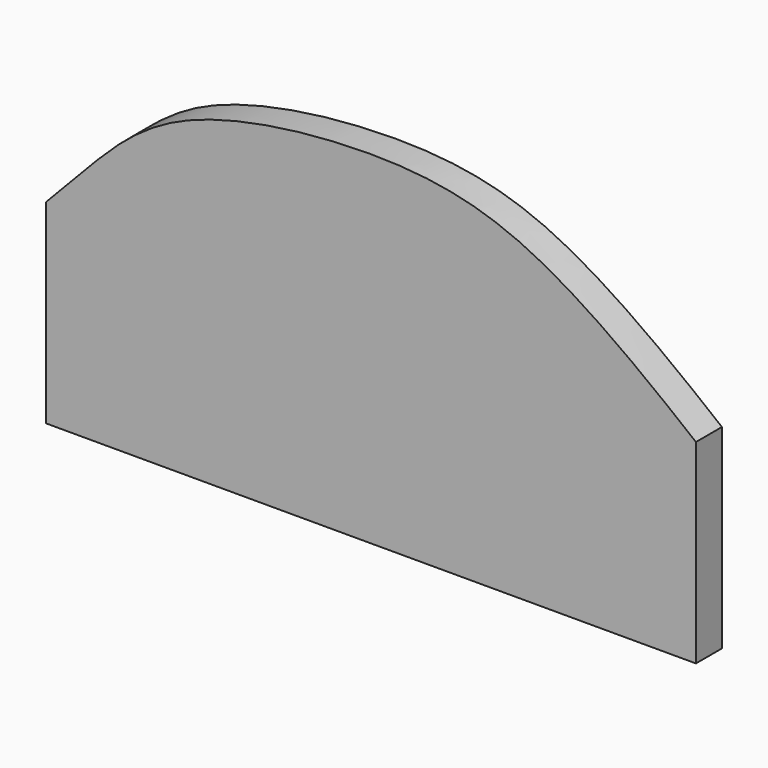
from build123d import *

# Parameters (mm, degrees)
F1_DEPTH = 6.35


with BuildPart() as f1:
    # F0 (on Front) → F1 (new body)
    with BuildSketch(Plane.XZ):
        with BuildLine():
            Line((-63.5, -38.1), (63.5, -38.1))
            Line((63.5, -38.1), (63.5, 0))
            add(Edge.make_bspline(
                [(-63.5, 0), (-60.67212487, 3.0032077004), (-54.227297491, 9.8476242046), (-38.4935463186, 25.5058577681), (0.6281666855, 30.5713039167), (28.1408073024, 25.8822175031), (51.7311119878, 9.4765375074), (60.0037451352, 2.8152524119), (63.5, 0)],
                knots=[0, 0, 0, 0, 0.1249399267, 0.2847425092, 0.498762547, 0.6847104917, 0.8667495031, 1, 1, 1, 1], degree=3))
            Line((-63.5, 0), (-63.5, -38.1))
        make_face()
    extrude(amount=F1_DEPTH)


solid = f1.part
